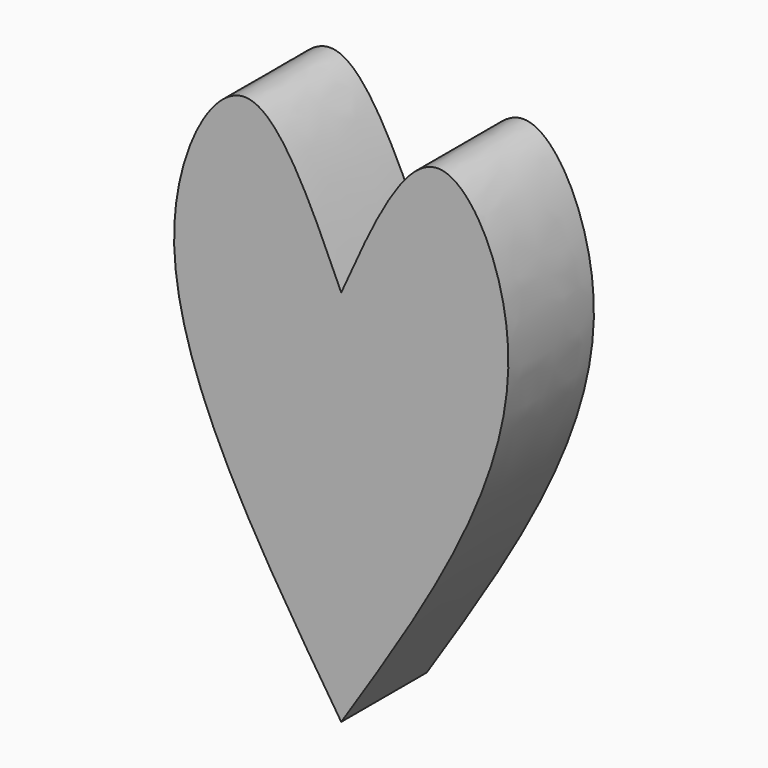
from build123d import *

# Parameters (mm, degrees)
F1_DEPTH = 5.08


with BuildPart() as f1:
    # F0 (on Front) → F1 (new body)
    with BuildSketch(Plane.XZ):
        with BuildLine():
            add(Edge.make_bspline(
                [(0, 16.8204726203), (1.5029023869, 20.1926711462), (4.4451183928, 26.7943883066), (10.5596723525, 15.0659398731), (4.0359001366, 5.055551181), (0, -1.1373273797)],
                knots=[0, 0, 0, 0, 0.2847963031, 0.5575426912, 1, 1, 1, 1], degree=3))
            add(Edge.make_bspline(
                [(0, 16.8204726203), (-1.5029023869, 20.1926711462), (-4.4451183928, 26.7943883066), (-10.5596723525, 15.0659398731), (-4.0359001366, 5.055551181), (0, -1.1373273797)],
                knots=[0, 0, 0, 0, 0.2847963031, 0.5575426912, 1, 1, 1, 1], degree=3))
        make_face()
    extrude(amount=F1_DEPTH)


solid = f1.part
